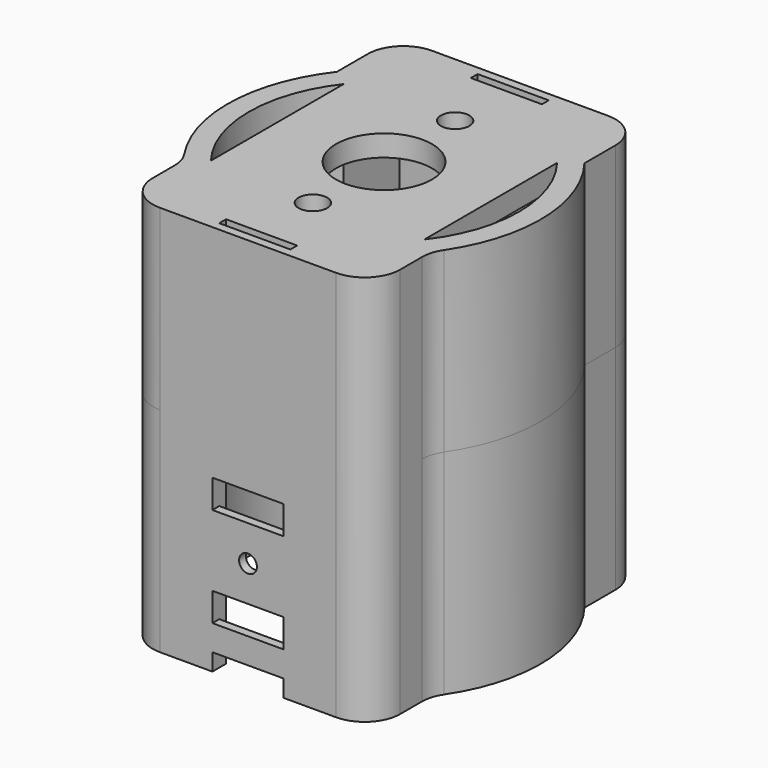
from build123d import *

# Parameters (mm, degrees)
F0_W     = 10
F0_H     = 1.2
F1_DEPTH = 30
F2_W     = 10
F2_H     = 4
F2_R     = 1.25
F3_DEPTH = 47.801
F4_DEPTH = 2.4
F5_R     = 5
F6_DEPTH = 25
F7_R     = 2
F7_R_2   = 6.75
F8_DEPTH = 3


# Not quite as in the source:
# - a feature names something its author has since deleted; it is built from what else it names


with BuildPart() as f1:
    # F0 (on Top) → F1 (new body)
    with BuildSketch(Plane.XY):
        with BuildLine():
            Line((15, -11.6619037897), (15, -21.5))
            Line((15, -21.5), (5, -21.5))
            Line((5, -21.5), (5, -22.7))
            Line((5, -22.7), (5, -23.9))
            Line((5, -23.9), (17.4, -23.9))
            Line((17.4, -23.9), (17.4, -13.462540622))
            ThreePointArc((17.4, -13.462540622), (22, 0), (17.4, 13.462540622))
            Line((17.4, 13.462540622), (17.4, 23.9))
            Line((17.4, 23.9), (5, 23.9))
            Line((5, 23.9), (5, 22.7))
            Line((5, 22.7), (5, 21.5))
            Line((5, 21.5), (15, 21.5))
            Line((15, 21.5), (15, 11.6619037897))
            ThreePointArc((15, 11.6619037897), (19, 0), (15, -11.6619037897))
        make_face()
        with Locations((0, 23.3)):
            Rectangle(F0_W, F0_H)
        with BuildLine():
            Line((-5, -23.9), (-5, -22.7))
            Line((-5, -22.7), (-5, -21.5))
            Line((-5, -21.5), (-15, -21.5))
            Line((-15, -21.5), (-15, -11.6619037897))
            ThreePointArc((-15, -11.6619037897), (-19, 0), (-15, 11.6619037897))
            Line((-15, 11.6619037897), (-15, 21.5))
            Line((-15, 21.5), (-5, 21.5))
            Line((-5, 21.5), (-5, 22.7))
            Line((-5, 22.7), (-5, 23.9))
            Line((-5, 23.9), (-17.4, 23.9))
            Line((-17.4, 23.9), (-17.4, 13.462540622))
            ThreePointArc((-17.4, 13.462540622), (-22, 0), (-17.4, -13.462540622))
            Line((-17.4, -13.462540622), (-17.4, -23.9))
            Line((-17.4, -23.9), (-5, -23.9))
        make_face()
        with Locations((0, -23.3)):
            Rectangle(F0_W, F0_H)
    extrude(amount=F1_DEPTH)

    # F2 (on face) → F3 (cut, through all)
    with BuildSketch(Plane.XZ.offset(23.9)):
        with Locations((0, 22)):
            Rectangle(F2_W, F2_H)
        with Locations((0, 8)):
            Rectangle(F2_W, F2_H)
        with Locations((0, 15)):
            Circle(F2_R)
    extrude(amount=-F3_DEPTH, mode=Mode.SUBTRACT)

    # F0 (on Top) → F4 (cut)
    with BuildSketch(Plane.XY):
        with Locations((0, 23.3)):
            Rectangle(F0_W, F0_H)
        with Locations((0, -23.3)):
            Rectangle(F0_W, F0_H)
    extrude(amount=F4_DEPTH, mode=Mode.SUBTRACT)

    # F5
    f5_edges = [f1.edges().sort_by_distance(p)[0] for p in [
        (-17.4, -23.9, 15),
        (17.4, -23.9, 15),
        (-17.4, -13.462541, 15),
        (-17.4, 23.9, 15),
        (17.4, 23.9, 15),
        (17.4, -13.462541, 15),
    ]]
    fillet(f5_edges, radius=F5_R)

    # F6 (add): a face of the model
    f6_faces = [f1.faces().sort_by_distance(p)[0] for p in [
        (16.7503200788, -16.9872408745, 30),
    ]]
    extrude(f6_faces, amount=F6_DEPTH)

    # F7 (on face) → F8 (join)
    with BuildSketch(Plane.XY.offset(55)):
        Polygon((-15, -11.6619037897), (-15, -21.5), (-5, -21.5), (5, -21.5), (15, -21.5), (15, -11.6619037897), (15, 11.6619037897), (15, 21.5), (5, 21.5), (-5, 21.5), (-15, 21.5), (-15, 11.6619037897), align=None)
        with Locations((0, -12.5)):
            Circle(F7_R, mode=Mode.SUBTRACT)
        Circle(F7_R_2, mode=Mode.SUBTRACT)
        with Locations((0, 12.5)):
            Circle(F7_R, mode=Mode.SUBTRACT)
    extrude(amount=-F8_DEPTH)


solid = f1.part
